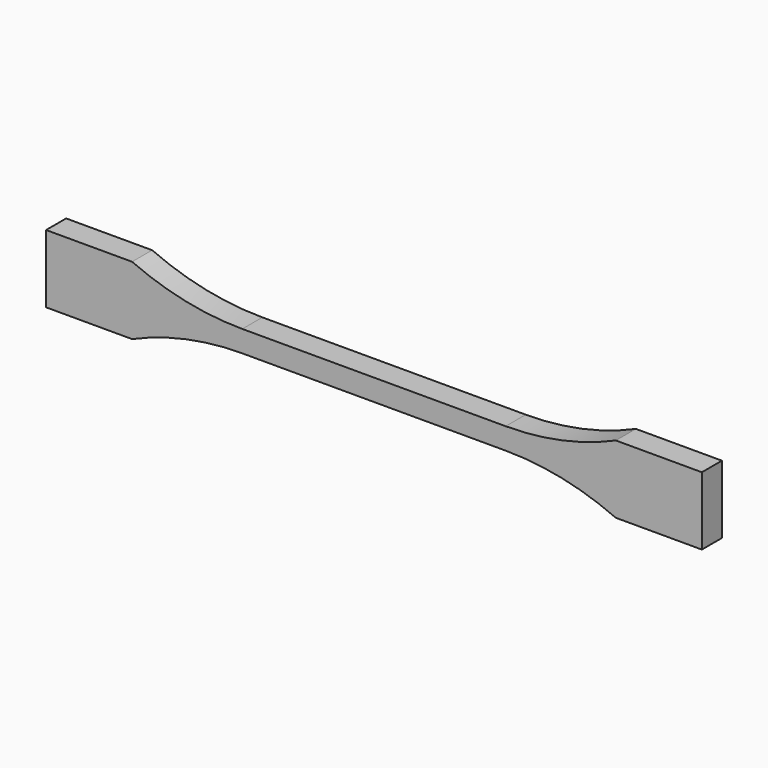
from build123d import *

# Parameters (mm, degrees)
F1_DEPTH = 7


# Not quite as in the source:
# - ends of sketch curves that miss each other by under 0.0002 mm in the source are joined


with BuildPart() as f1:
    # F0 (on Front) → F1 (new body)
    with BuildSketch(Plane.XZ):
        with BuildLine():
            Line((36.7469513706, 3), (1.8211e-06, 3))
            Line((1.8211e-06, 3), (-36.7469513706, 3))
            ThreePointArc((-36.7469513706, 3), (-52.4631850161, 4.6427542199), (-67.5, 9.5))
            Line((-67.5, 9.5), (-91.5, 9.5))
            Line((-91.5, 9.5), (-91.5, 0))
            Line((-91.5, 0), (-91.5, -9.5))
            Line((-91.5, -9.5), (-67.5, -9.5))
            ThreePointArc((-67.5, -9.5), (-52.4631850161, -4.6427542199), (-36.7469513706, -3))
            Line((-36.7469513706, -3), (-1.8211e-06, -3))
            Line((-1.8211e-06, -3), (36.7469513706, -3))
            ThreePointArc((36.7469513706, -3), (52.4631850161, -4.6427542199), (67.5, -9.5))
            Line((67.5, -9.5), (91.5, -9.5))
            Line((91.5, -9.5), (91.5, 0))
            Line((91.5, 0), (91.5, 9.5))
            Line((91.5, 9.5), (67.5, 9.5))
            ThreePointArc((67.5, 9.5), (52.4631850161, 4.6427542199), (36.7469513706, 3))
        make_face()
    extrude(amount=F1_DEPTH)


solid = f1.part
